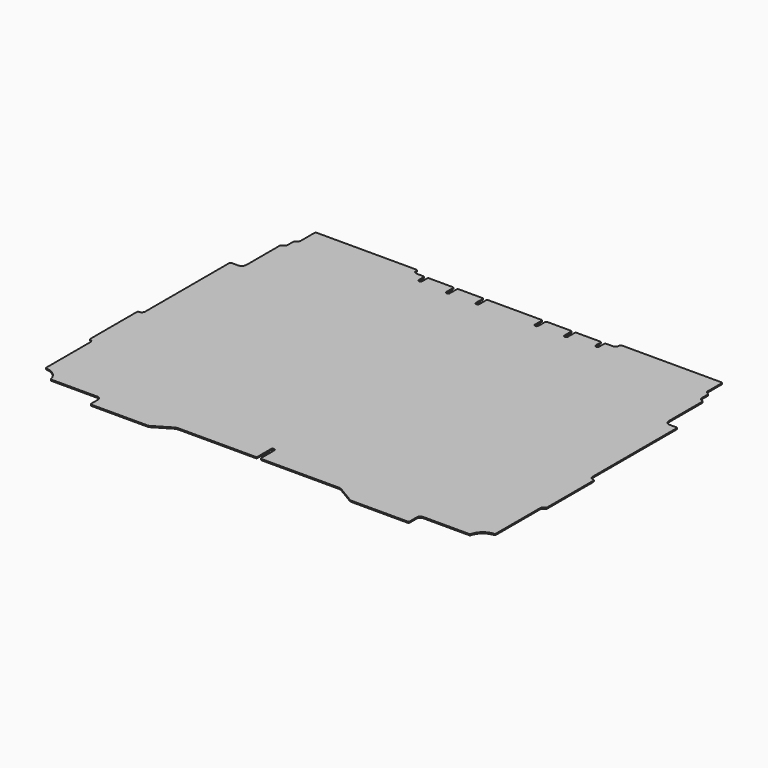
from build123d import *

# Parameters (mm, degrees)
F1_DEPTH = 1
F2_R     = 1
F3_R     = 5


# Not quite as in the source:
# - ends of sketch curves that miss each other by under 0.0002 mm in the source are joined


with BuildPart() as f1:
    # F0 (on Top) → F1 (new body)
    with BuildSketch(Plane.XY):
        with BuildLine():
            ThreePointArc((-93.3991712707, -123.0276243094), (-85.1530297199, -125.9847384402), (-80.6653146424, -133.5082873263))
            Line((-80.6653146424, -133.5082873263), (-40.9958563536, -133.5082872928))
            ThreePointArc((-40.9958563536, -133.5082872928), (-38.8784426773, -134.3853487547), (-38.0013812155, -136.5027624309))
            Line((-38.0013812155, -136.5027624309), (-38.0013812155, -144.9871086556))
            Line((-38.0013812155, -144.9871086556), (11.4074585635, -144.9871086556))
            Line((11.4074585635, -144.9871086556), (25.9643957459, -136.3439274843))
            ThreePointArc((25.9643957459, -136.3439274843), (27.4366380226, -135.7182454478), (29.0219874328, -135.5046040516))
            Line((29.0219874328, -135.5046040516), (95.2527624309, -135.5046040516))
            Line((95.2527624309, -135.5046040516), (95.2527624309, -120.532228361))
            ThreePointArc((95.2527624309, -120.532228361), (95.6912931619, -119.4735215228), (96.75, -119.0349907919))
            Line((96.75, -119.0349907919), (96.75, 135.4953959484))
            Line((96.75, 135.4953959484), (73.2932780847, 135.4953959484))
            Line((73.2932780847, 135.4953959484), (73.2932780847, 127.5101289134))
            ThreePointArc((73.2932780847, 127.5101289134), (71.7960405157, 126.0128913444), (70.2988029466, 127.5101289134))
            Line((70.2988029466, 127.5101289134), (70.2988029466, 135.4953959484))
            Line((70.2988029466, 135.4953959484), (48.3393186004, 135.4953959484))
            Line((48.3393186004, 135.4953959484), (48.3393186004, 127.5101289134))
            ThreePointArc((48.3393186004, 127.5101289134), (46.8420810313, 126.0128913444), (45.3448434622, 127.5101289134))
            Line((45.3448434622, 127.5101289134), (45.3448434622, 135.4953959484))
            Line((45.3448434622, 135.4953959484), (23.3872, 135.4953959484))
            Line((23.3872, 135.4953959484), (23.3872, 129.5064456722))
            ThreePointArc((23.3872, 129.5064456722), (21.889965, 128.0092106722), (20.39273, 129.5064456722))
            Line((20.39273, 129.5064456722), (20.39273, 135.4953959484))
            Line((20.39273, 135.4953959484), (13.902854512, 135.4953959484))
            ThreePointArc((13.902854512, 135.4953959484), (11.7854408357, 136.3724574103), (10.9083793738, 138.4898710866))
            Line((10.9083793738, 138.4898710866), (10.9083793738, 139.9871086556))
            Line((10.9083793738, 139.9871086556), (-75.432320442, 139.9871086556))
            Line((-75.432320442, 139.9871086556), (-75.432320442, 124.5156537753))
            ThreePointArc((-75.432320442, 124.5156537753), (-76.3093819039, 122.3982400991), (-78.4267955801, 121.5211786372))
            Line((-78.4267955801, 121.5211786372), (-78.4267955801, 114.5340699816))
            ThreePointArc((-78.4267955801, 114.5340699816), (-79.303857042, 112.4166563053), (-81.4212707182, 111.5395948435))
            Line((-81.4212707182, 111.5395948435), (-81.9203499079, 111.5395948435))
            Line((-81.9203499079, 111.5395948435), (-81.9203499079, 75.1068139963))
            ThreePointArc((-81.9203499079, 75.1068139963), (-83.0897651904, 72.2835957613), (-85.9129834254, 71.1141804788))
            Line((-85.9129834254, 71.1141804788), (-92.4010128913, 71.1141804788))
            Line((-92.4010128913, 71.1141804788), (-92.4010128913, -18.7200736648))
            ThreePointArc((-92.4010128913, -18.7200736648), (-93.2780743532, -20.8374873411), (-95.3954880295, -21.7145488029))
            Line((-95.3954880295, -21.7145488029), (-96.3936464088, -21.7145488029))
            Line((-96.3936464088, -21.7145488029), (-96.3936464088, -72.620626151))
            ThreePointArc((-96.3936464088, -72.620626151), (-94.2762327326, -73.4976876129), (-93.3991712707, -75.6151012891))
            Line((-93.3991712707, -75.6151012891), (-93.3991712707, -123.0276243094))
        make_face()
        with BuildLine():
            Line((96.75, 135.4953959484), (96.75, -119.0349907919))
            ThreePointArc((96.75, -119.0349907919), (97.8087068381, -119.4735215228), (98.2472375691, -120.532228361))
            Line((98.2472375691, -120.532228361), (98.2472375691, -135.5046040516))
            Line((98.2472375691, -135.5046040516), (164.4780125672, -135.5046040516))
            ThreePointArc((164.4780125672, -135.5046040516), (166.0633619774, -135.7182454478), (167.5356043334, -136.3439273508))
            Line((167.5356043334, -136.3439273508), (182.0925414365, -144.9871086556))
            Line((182.0925414365, -144.9871086556), (231.5013812155, -144.9871086556))
            Line((231.5013812155, -144.9871086556), (231.5013812155, -136.5027624309))
            ThreePointArc((231.5013812155, -136.5027624309), (232.3784426773, -134.3853487547), (234.4958563536, -133.5082872928))
            Line((234.4958563536, -133.5082872928), (274.1653144715, -133.5082872928))
            ThreePointArc((274.1653144715, -133.5082872928), (278.6530297199, -125.9847384402), (286.8991712707, -123.0276243094))
            Line((286.8991712707, -123.0276243094), (286.8991712707, -75.6151012891))
            ThreePointArc((286.8991712707, -75.6151012891), (287.7762327326, -73.4976876129), (289.8936464088, -72.620626151))
            Line((289.8936464088, -72.620626151), (289.8936464088, -21.7145488029))
            Line((289.8936464088, -21.7145488029), (288.8954880295, -21.7145488029))
            ThreePointArc((288.8954880295, -21.7145488029), (286.7780743532, -20.8374873411), (285.9010128913, -18.7200736648))
            Line((285.9010128913, -18.7200736648), (285.9010128913, 71.1141804788))
            Line((285.9010128913, 71.1141804788), (279.4129834254, 71.1141804788))
            ThreePointArc((279.4129834254, 71.1141804788), (276.5897651904, 72.2835957613), (275.4203499079, 75.1068139963))
            Line((275.4203499079, 75.1068139963), (275.4203499079, 111.5395948435))
            Line((275.4203499079, 111.5395948435), (274.9212707182, 111.5395948435))
            ThreePointArc((274.9212707182, 111.5395948435), (272.803857042, 112.4166563053), (271.9267955801, 114.5340699816))
            Line((271.9267955801, 114.5340699816), (271.9267955801, 121.5211786372))
            ThreePointArc((271.9267955801, 121.5211786372), (269.8093819039, 122.3982400991), (268.932320442, 124.5156537753))
            Line((268.932320442, 124.5156537753), (268.932320442, 139.9871086556))
            Line((268.932320442, 139.9871086556), (182.5916206262, 139.9871086556))
            Line((182.5916206262, 139.9871086556), (182.5916206262, 138.4898710866))
            ThreePointArc((182.5916206262, 138.4898710866), (181.7145591643, 136.3724574103), (179.597145488, 135.4953959484))
            Line((179.597145488, 135.4953959484), (173.10727, 135.4953959484))
            Line((173.10727, 135.4953959484), (173.10727, 129.5064456722))
            ThreePointArc((173.10727, 129.5064456722), (171.610035, 128.0092106722), (170.1128, 129.5064456722))
            Line((170.1128, 129.5064456722), (170.1128, 135.4953959484))
            Line((170.1128, 135.4953959484), (148.1551565378, 135.4953959484))
            Line((148.1551565378, 135.4953959484), (148.1551565378, 127.5101289134))
            ThreePointArc((148.1551565378, 127.5101289134), (146.6579189687, 126.0128913444), (145.1606813996, 127.5101289134))
            Line((145.1606813996, 127.5101289134), (145.1606813996, 135.4953959484))
            Line((145.1606813996, 135.4953959484), (123.2011970534, 135.4953959484))
            Line((123.2011970534, 135.4953959484), (123.2011970534, 127.5101289134))
            ThreePointArc((123.2011970534, 127.5101289134), (121.7039594843, 126.0128913444), (120.2067219153, 127.5101289134))
            Line((120.2067219153, 127.5101289134), (120.2067219153, 135.4953959484))
            Line((120.2067219153, 135.4953959484), (96.75, 135.4953959484))
        make_face()
    extrude(amount=F1_DEPTH)

    # F2
    f2_edges = [f1.edges().sort_by_distance(p)[0] for p in [
        (-38.001381, -144.987109, 0.5),
        (-80.665315, -133.508287, 0.5),
        (-93.399171, -123.027624, 0.5),
        (-96.393646, -72.620626, 0.5),
        (-96.393646, -21.714549, 0.5),
        (-92.401013, 71.11418, 0.5),
        (-81.92035, 111.539595, 0.5),
        (-78.426796, 121.521179, 0.5),
        (-75.43232, 139.987109, 0.5),
        (10.908379, 139.987109, 0.5),
        (20.39273, 135.495396, 0.5),
        (23.3872, 135.495396, 0.5),
        (45.344843, 135.495396, 0.5),
        (48.339319, 135.495396, 0.5),
        (70.298803, 135.495396, 0.5),
        (73.293278, 135.495396, 0.5),
        (120.206722, 135.495396, 0.5),
        (123.201197, 135.495396, 0.5),
        (145.160681, 135.495396, 0.5),
        (148.155157, 135.495396, 0.5),
        (170.1128, 135.495396, 0.5),
        (173.10727, 135.495396, 0.5),
        (182.591621, 139.987109, 0.5),
        (268.93232, 139.987109, 0.5),
        (271.926796, 121.521179, 0.5),
        (275.42035, 111.539595, 0.5),
        (285.901013, 71.11418, 0.5),
        (289.893646, -21.714549, 0.5),
        (289.893646, -72.620626, 0.5),
        (286.899171, -123.027624, 0.5),
        (274.165314, -133.508287, 0.5),
        (231.501381, -144.987109, 0.5),
        (98.247238, -135.504604, 0.5),
        (95.252762, -135.504604, 0.5),
    ]]
    fillet(f2_edges, radius=F2_R)

    # F3
    f3_edges = [f1.edges().sort_by_distance(p)[0] for p in [
        (182.092541, -144.987109, 0.5),
        (11.407459, -144.987109, 0.5),
    ]]
    fillet(f3_edges, radius=F3_R)


solid = f1.part
